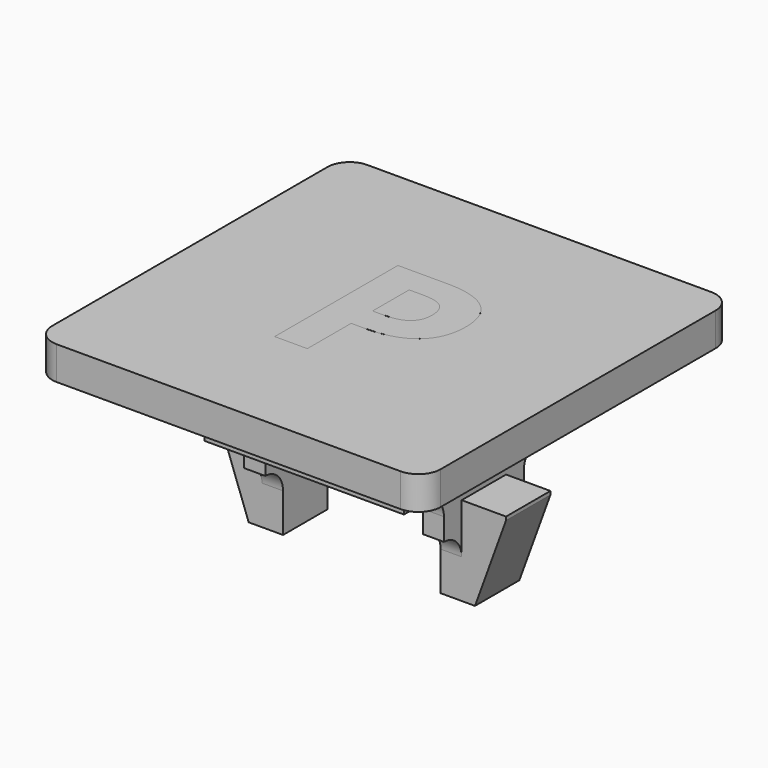
from build123d import *

# Parameters (mm, degrees)
F0_DEPTH      = 1.5
F1_W          = 9
F1_H          = 10
F1_W_2        = 7.1
F1_H_2        = 8.4
F2_DEPTH      = 5
F3_W          = 2.5
F3_H          = 1.25
F3_H_2        = 2.75
F4_DEPTH      = 2
F4_DEPTH_BACK = 0.95
F5_SIZE2      = 3.8464683872
F5_SIZE       = 1.4
F6_START      = -8.05
F3_H_3        = 4
F6_DEPTH      = 2.95
F7_SIZE2      = 3.8464683872
F7_SIZE       = 1.4
F8_R          = 1
F14_TEXT_SIZE = 9.7222222222
F9_DEPTH      = 1.5
F11_DEPTH     = 2
F12_DEPTH     = 2
F13_R         = 1


# Not quite as in the source:
# - Text() gives the source's letters only with a copy of the font that has no kerning and outlines rounded to 1/6400 em; it was checked with that copy


with BuildPart() as f0:
    # F14 (on Top) → F0 (new body)
    with BuildSketch(Plane.XY):
        with BuildLine():
            Line((7.75, 8.75), (-7.75, 8.75))
            ThreePointArc((-7.75, 8.75), (-8.4571067812, 8.4571067812), (-8.75, 7.75))
            Line((-8.75, 7.75), (-8.75, -7.75))
            ThreePointArc((-8.75, -7.75), (-8.4571067812, -8.4571067812), (-7.75, -8.75))
            Line((-7.75, -8.75), (7.75, -8.75))
            ThreePointArc((7.75, -8.75), (8.4571067812, -8.4571067812), (8.75, -7.75))
            Line((8.75, -7.75), (8.75, 7.75))
            ThreePointArc((8.75, 7.75), (8.4571067812, 8.4571067812), (7.75, 8.75))
        make_face()
        with BuildLine():
            add(Edge.make_bspline(
                [(2.0107421875, 2.8969184028), (2.6677517361, 2.3530815972), (2.6677517361, 1.2760416667)],
                knots=[0, 0, 0, 1, 1, 1], degree=2))
            add(Edge.make_bspline(
                [(2.6677517361, 1.2760416667), (2.6677517361, 0.1549479167), (1.9674479167, -0.4382595486)],
                knots=[0, 0, 0, 1, 1, 1], degree=2))
            add(Edge.make_bspline(
                [(1.9674479167, -0.4382595486), (1.2671440972, -1.0314670139), (-0.0240885417, -1.0314670139)],
                knots=[0, 0, 0, 1, 1, 1], degree=2))
            Line((-0.0240885417, -1.0314670139), (-0.6545138889, -1.0314670139))
            Line((-0.6545138889, -1.0314670139), (-0.6545138889, -3.5))
            Line((-0.6545138889, -3.5), (-2.1265190972, -3.5))
            Line((-2.1265190972, -3.5), (-2.1265190972, 3.4407552083))
            Line((-2.1265190972, 3.4407552083), (0.08984375, 3.4407552083))
            add(Edge.make_bspline(
                [(0.08984375, 3.4407552083), (1.3537326389, 3.4407552083), (2.0107421875, 2.8969184028)],
                knots=[0, 0, 0, 1, 1, 1], degree=2))
        make_face(mode=Mode.SUBTRACT)
    extrude(amount=F0_DEPTH)

    # F1 (on face) → F2 (join)
    with BuildSketch(Plane(origin=(0, 0, 0), x_dir=(1, 0, 0), z_dir=(0, 0, -1))):
        with Locations((0, -0.5)):
            Rectangle(F1_W, F1_H)
        with Locations((0, -0.5)):
            Rectangle(F1_W_2, F1_H_2, mode=Mode.SUBTRACT)
    extrude(amount=F2_DEPTH)

    # F3 (on face) → F4 (join, two sides)
    with BuildSketch(Plane.YZ.offset(4.5)) as f4_sk:
        with Locations((0, -4.375)):
            Rectangle(F3_W, F3_H)
        with Locations((0, -6.375)):
            Rectangle(F3_W, F3_H_2)
    extrude(amount=F4_DEPTH)
    extrude(f4_sk.sketch, amount=-F4_DEPTH_BACK)

    # F5
    f5_edges = [f0.edges().sort_by_distance(p)[0] for p in [
        (6.5, 0, -7.75),
    ]]
    f5_side = f0.faces().sort_by_distance((5.025, 0, -7.75))[0]
    chamfer(f5_edges, length=F5_SIZE, length2=F5_SIZE2, reference=f5_side)

    # F3 (on face) → F6 (join)
    with BuildSketch(Plane.YZ.offset(4.5).offset(F6_START)):
        with Locations((0, -5.75)):
            Rectangle(F3_W, F3_H_3)
    extrude(amount=-F6_DEPTH)

    # F7
    f7_edges = [f0.edges().sort_by_distance(p)[0] for p in [
        (-6.5, 0, -7.75),
    ]]
    f7_side = f0.faces().sort_by_distance((-5.025, 0, -7.75))[0]
    chamfer(f7_edges, length=F7_SIZE, length2=F7_SIZE2, reference=f7_side)

    # F8
    f8_edges = [f0.edges().sort_by_distance(p)[0] for p in [
        (-4.025, -1.25, -5),
        (-4.025, 1.25, -5),
        (4.025, -1.25, -5),
        (4.025, 1.25, -5),
    ]]
    fillet(f8_edges, radius=F8_R)

    # F12 (cut): faces of the model
    f12_faces = [f0.faces().sort_by_distance(p)[0] for p in [
        (-3.645688296, 3.475, -5),
        (0, -3.7886614766, -5),
    ]]
    extrude(f12_faces, amount=-F12_DEPTH, mode=Mode.SUBTRACT)

    # F13
    f13_edges = [f0.edges().sort_by_distance(p)[0] for p in [
        (-4.025, 2.25, -3),
        (4.025, 2.25, -3),
        (4.025, -2.25, -3),
        (-4.025, -2.25, -3),
    ]]
    fillet(f13_edges, radius=F13_R)


with BuildPart() as f0b:
    # F14 (on Top) → F0, piece 2 (new body)
    with BuildSketch(Plane.XY):
        with BuildLine():
            Line((-0.6545138889, 2.2345920139), (-0.6545138889, 0.1746961806))
            Line((-0.6545138889, 0.1746961806), (-0.169921875, 0.1746961806))
            add(Edge.make_bspline(
                [(-0.169921875, 0.1746961806), (0.5075954861, 0.1746961806), (0.8448350694, 0.4428168403)],
                knots=[0, 0, 0, 1, 1, 1], degree=2))
            add(Edge.make_bspline(
                [(0.8448350694, 0.4428168403), (1.1820746528, 0.7109375), (1.1820746528, 1.2228732639)],
                knots=[0, 0, 0, 1, 1, 1], degree=2))
            add(Edge.make_bspline(
                [(1.1820746528, 1.2228732639), (1.1820746528, 1.7408854167), (0.8995225694, 1.9877387153)],
                knots=[0, 0, 0, 1, 1, 1], degree=2))
            add(Edge.make_bspline(
                [(0.8995225694, 1.9877387153), (0.6169704861, 2.2345920139), (0.0138888889, 2.2345920139)],
                knots=[0, 0, 0, 1, 1, 1], degree=2))
            Line((0.0138888889, 2.2345920139), (-0.6545138889, 2.2345920139))
        make_face()
    extrude(amount=F0_DEPTH)


with BuildPart() as f9:
    # F14 (on Top) → F9 (new body, through all)
    with BuildSketch(Plane.XY):
        with Locations((-3, -3.5)):
            Text('P', F14_TEXT_SIZE, font='Open Sans', font_style=FontStyle.BOLD, text_align=(TextAlign.LEFT, TextAlign.BOTTOM))
    extrude(amount=F9_DEPTH)

    # F10 (on face) → F11 (join)
    with BuildSketch(Plane(origin=(0, 0, 0), x_dir=(1, 0, 0), z_dir=(0, 0, -1))):
        with BuildLine():
            add(Edge.make_bspline(
                [(2.5466790527, -2.1024799736), (2.6677517361, -1.7383897356), (2.6677517361, -1.2760416667)],
                knots=[0.5707233726, 0.5707233726, 0.5707233726, 1, 1, 1], degree=2))
            ThreePointArc((2.5466790527, -2.1024799736), (2.8434984759, -1.7490662241), (2.95, -1.3))
            Line((2.95, -1.3), (2.95, 0.7))
            ThreePointArc((2.95, 0.7), (2.6571067812, 1.4071067812), (1.95, 1.7))
            Line((1.95, 1.7), (-0.6545138889, 1.7))
            Line((-0.6545138889, 1.7), (-0.6545138889, 1.0314670139))
            Line((-0.6545138889, 1.0314670139), (-0.0240885417, 1.0314670139))
            add(Edge.make_bspline(
                [(1.9674479167, 0.4382595486), (1.2671440972, 1.0314670139), (-0.0240885417, 1.0314670139)],
                knots=[0, 0, 0, 1, 1, 1], degree=2))
            add(Edge.make_bspline(
                [(2.6677517361, -1.2760416667), (2.6677517361, -0.1549479167), (1.9674479167, 0.4382595486)],
                knots=[0, 0, 0, 1, 1, 1], degree=2))
        make_face()
        with BuildLine():
            ThreePointArc((-3.05, -1.3), (-2.7836617399, -1.9795148647), (-2.1265190972, -2.2970681159))
            Line((-2.1265190972, -2.2970681159), (-2.1265190972, 1.6970681159))
            ThreePointArc((-2.1265190972, 1.6970681159), (-2.7836617399, 1.3795148647), (-3.05, 0.7))
            Line((-3.05, 0.7), (-3.05, -1.3))
        make_face()
        with BuildLine():
            Line((-2.05, -2.3), (1.95, -2.3))
            ThreePointArc((1.95, -2.3), (2.264261059, -2.2493366035), (2.5466790527, -2.1024799736))
            add(Edge.make_bspline(
                [(2.5466790527, -2.1024799736), (2.6677517361, -1.7383897356), (2.6677517361, -1.2760416667)],
                knots=[0.5707233726, 0.5707233726, 0.5707233726, 1, 1, 1], degree=2))
            add(Edge.make_bspline(
                [(2.6677517361, -1.2760416667), (2.6677517361, -0.1549479167), (1.9674479167, 0.4382595486)],
                knots=[0, 0, 0, 1, 1, 1], degree=2))
            add(Edge.make_bspline(
                [(1.9674479167, 0.4382595486), (1.2671440972, 1.0314670139), (-0.0240885417, 1.0314670139)],
                knots=[0, 0, 0, 1, 1, 1], degree=2))
            Line((-0.0240885417, 1.0314670139), (-0.6545138889, 1.0314670139))
            Line((-0.6545138889, 1.0314670139), (-0.6545138889, 1.7))
            Line((-0.6545138889, 1.7), (-2.05, 1.7))
            ThreePointArc((-2.05, 1.7), (-2.0882876226, 1.6992667602), (-2.1265190972, 1.6970681159))
            Line((-2.1265190972, 1.6970681159), (-2.1265190972, -2.2970681159))
            ThreePointArc((-2.1265190972, -2.2970681159), (-2.0882876226, -2.2992667602), (-2.05, -2.3))
        make_face()
    extrude(amount=F11_DEPTH)


solid = Compound([f0.part, f0b.part, f9.part])
